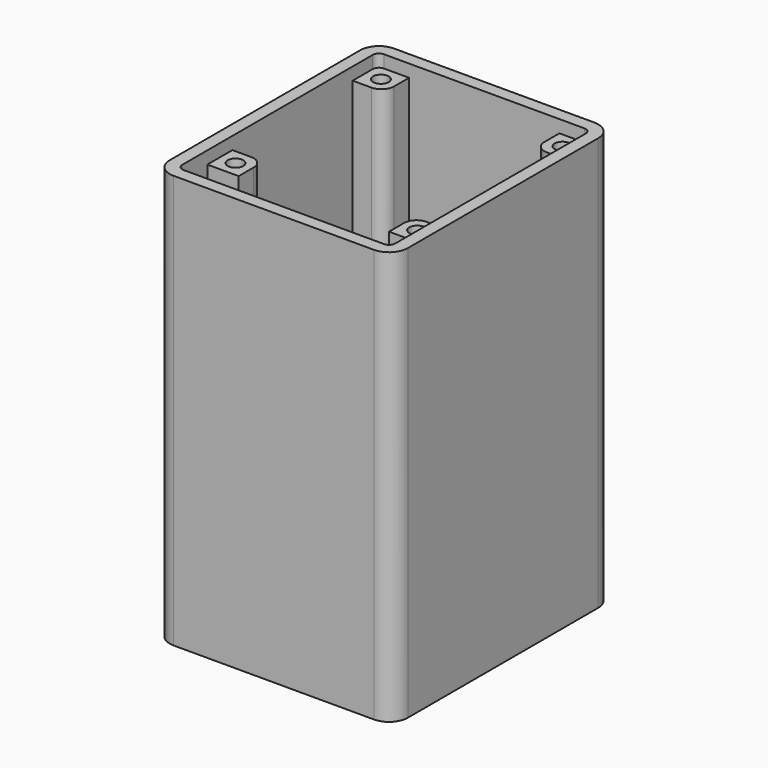
from build123d import *

# Parameters (mm, degrees)
F1_DEPTH     = 66
F2_T         = -2
F5_DEPTH     = 25
F6_R         = 1.25
F7_DEPTH     = 10
F8_TEXT_SIZE = 11.1111111111
F9_DEPTH     = 1


# Not quite as in the source:
# - Text() gives the source's letters only with a copy of the font that has no kerning and outlines rounded to 1/6400 em; it was checked with that copy


with BuildPart() as f1:
    # F0 (on Top) → F1 (new body)
    with BuildSketch(Plane.XY):
        with BuildLine():
            Line((16, 22), (-16, 22))
            ThreePointArc((-16, 22), (-18.1213203436, 21.1213203436), (-19, 19))
            Line((-19, 19), (-19, -19))
            ThreePointArc((-19, -19), (-18.1213203436, -21.1213203436), (-16, -22))
            Line((-16, -22), (16, -22))
            ThreePointArc((16, -22), (18.1213203436, -21.1213203436), (19, -19))
            Line((19, -19), (19, 19))
            ThreePointArc((19, 19), (18.1213203436, 21.1213203436), (16, 22))
        make_face()
    extrude(amount=F1_DEPTH)

    # F2
    f2_openings = [f1.faces().sort_by_distance(p)[0] for p in [
        (0, 0, 66),
    ]]
    offset(amount=F2_T, openings=f2_openings)

    # F4 (on offset) → F5 (join)
    with BuildSketch(Plane.XY.offset(64)):
        with BuildLine():
            Line((-12, 20), (-17, 20))
            Line((-17, 20), (-17, 15))
            Line((-17, 15), (-14, 15))
            ThreePointArc((-14, 15), (-12.5857864376, 15.5857864376), (-12, 17))
            Line((-12, 17), (-12, 20))
        make_face()
        with BuildLine():
            Line((17, 20), (12, 20))
            Line((12, 20), (12, 17))
            ThreePointArc((12, 17), (12.5857864376, 15.5857864376), (14, 15))
            Line((14, 15), (17, 15))
            Line((17, 15), (17, 20))
        make_face()
        with BuildLine():
            Line((-14, -9), (-17, -9))
            Line((-17, -9), (-17, -14))
            Line((-17, -14), (-12, -14))
            Line((-12, -14), (-12, -11))
            ThreePointArc((-12, -11), (-12.5857864376, -9.5857864376), (-14, -9))
        make_face()
        with BuildLine():
            Line((17, -14), (17, -9))
            Line((17, -9), (14, -9))
            ThreePointArc((14, -9), (12.5857864376, -9.5857864376), (12, -11))
            Line((12, -11), (12, -14))
            Line((12, -14), (17, -14))
        make_face()
    extrude(amount=-F5_DEPTH)

    # F6 (on face) → F7 (cut)
    with BuildSketch(Plane.XY.offset(64)):
        with Locations((-14.5, 17.5)):
            Circle(F6_R)
        with Locations((14.5, 17.5)):
            Circle(F6_R)
        with Locations((-14.5, -11.5)):
            Circle(F6_R)
        with Locations((14.5, -11.5)):
            Circle(F6_R)
    extrude(amount=-F7_DEPTH, mode=Mode.SUBTRACT)

    # F8 (on face) → F9 (join)
    with BuildSketch(Plane(origin=(-19, 0, 0), x_dir=(0, -1, 0), z_dir=(-1, 0, 0))):
        with Locations(Location((0, 4.6992456019), (0, 0, 90))):
            Text('PREDIKTAS', F8_TEXT_SIZE, font='Open Sans', text_align=(TextAlign.LEFT, TextAlign.BOTTOM))
    extrude(amount=F9_DEPTH)


solid = f1.part
